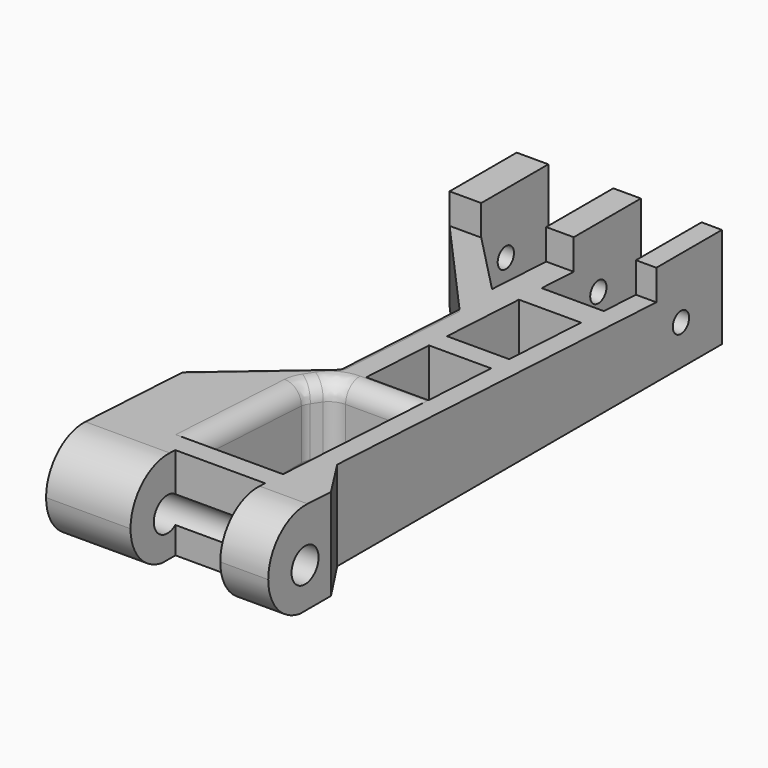
from build123d import *

# Parameters (mm, degrees)
F0_W     = 9.4565711915
F0_H     = 13.6675285175
F1_DEPTH = 15.3
F2_W     = 109.1410517693
F2_H     = 22.5323475897
F3_DEPTH = 77
F4_R     = 2.5676865252
F5_DEPTH = 65.4
F6_R     = 1.5468397632
F7_DEPTH = 54.6
F8_R     = 2.6556349186
F9_R     = 1
F10_R    = 0.0237853743


with BuildPart() as f1:
    # F0 (on Top) → F1 (new body)
    with BuildSketch(Plane.XY):
        Polygon((-40.6965725124, 44.3279668689), (-43.8004508615, 44.3550609052), (-43.8004508615, 25.7457569242), (-53.257022053, 25.7457569242), (-53.257022053, 44.6070879698), (-57.4438385665, 44.6070879698), (-57.4438385665, 21.5618759394), (-67.321151495, 31.8517945707), (-67.321151495, 44.6070879698), (-72.1341744065, 44.6070879698), (-72.1341744065, 31.8517945707), (-57.4438385665, 15.2993714437), (-57.4438385665, -7.5885597616), (-70.2834129333, -20.1490093023), (-70.2834129333, -50.7155247033), (-57.4438385665, -50.7155247033), (-57.4438385665, -38.6135876179), (-43.8004508615, -38.6135876179), (-43.8004508615, -50.7155247033), (-36.5097559988, -50.7155247033), (-36.5097559988, -35.2215506136), (-40.6965725124, -28.8017634302), align=None)
        Polygon((-43.8004508615, -10.5956946412), (-43.8004508615, -35.2215506136), (-57.4438385665, -35.2215506136), (-57.4438385665, -14.0083450824), (-55.5479216548, -10.5956946412), align=None, mode=Mode.SUBTRACT)
        Polygon((-49.6741862581, -7.5885597616), (-53.257022053, -7.5885597616), (-53.257022053, 4.3360902928), (-49.6741862581, 4.3360902928), (-43.8004508615, 4.3360902928), (-43.8004508615, -7.5885597616), align=None, mode=Mode.SUBTRACT)
        with Locations((-48.5287364572, 14.5968659781)):
            Rectangle(F0_W, F0_H, mode=Mode.SUBTRACT)
    extrude(amount=F1_DEPTH)

    # F2 (on face) → F3 (cut)
    with BuildSketch(Plane(origin=(-72.1341744065, 0, 0), x_dir=(0, -1, 0), z_dir=(-1, 0, 0))):
        with Locations((3.7736594677, 6.6085606813)):
            Rectangle(F2_W, F2_H)
        with BuildLine():
            ThreePointArc((39.6816573, 14.1380049634), (44.9345471885, 12.1822751735), (47.1420204778, 7.0301112719))
            ThreePointArc((47.1420204778, 7.0301112719), (44.6510850499, 1.622031227), (38.9221144813, 0))
            Line((38.9221144813, 0), (-31.8517945707, 0))
            Line((-31.8517945707, 0), (-37.1405081916, 0))
            ThreePointArc((-37.1405081916, 0), (-38.2294412702, -0.1143932508), (-39.3183743488, 0))
            Line((-39.3183743488, 0), (-44.6070879698, 0))
            Line((-44.6070879698, 0), (-44.6070879698, 15.3))
            Line((-44.6070879698, 15.3), (-31.8517945707, 15.3))
            Line((-31.8517945707, 15.3), (-31.8517945707, 10.6745666141))
            Line((-31.8517945707, 10.6745666141), (39.6816573, 14.1380049634))
        make_face(mode=Mode.SUBTRACT)
    extrude(amount=-F3_DEPTH, mode=Mode.SUBTRACT)

    # F4 (on face) → F5 (cut)
    with BuildSketch(Plane(origin=(-72.1341744065, 0, 0), x_dir=(0, -1, 0), z_dir=(-1, 0, 0))):
        with Locations((40.1412695646, 6.1273775063)):
            Circle(F4_R)
    extrude(amount=-F5_DEPTH, mode=Mode.SUBTRACT)

    # F6 (on face) → F7 (cut)
    with BuildSketch(Plane(origin=(-72.1341744065, 0, 0), x_dir=(0, -1, 0), z_dir=(-1, 0, 0))):
        with Locations((-36.5287549794, 6.0891942121)):
            Circle(F6_R)
    extrude(amount=-F7_DEPTH, mode=Mode.SUBTRACT)

    # F8
    f8_edges = [f1.edges().sort_by_distance(p)[0] for p in [
        (-56.49588, -12.30202, 0),
        (-55.547922, -10.595695, 6.364874),
        (-56.49588, -12.30202, 12.812364),
        (-57.443839, -14.008345, 6.44749),
        (-49.674186, -10.595695, 0),
        (-57.443839, -24.614948, 0),
        (-49.674186, -10.595695, 12.729749),
        (-57.443839, -24.614948, 13.408519),
    ]]
    fillet(f8_edges, radius=F8_R)

    # F9
    f9_edges = [f1.edges().sort_by_distance(p)[0] for p in [
        (-63.863626, -13.868785, 0),
        (-70.283413, -20.149009, 6.596146),
        (-63.863626, -13.868785, 12.888222),
        (-57.443839, -7.58856, 6.292076),
        (-57.443839, 3.855406, 0),
        (-57.443839, 3.855406, 12.030069),
    ]]
    fillet(f9_edges, radius=F9_R)

    # F10
    f10_edges = [f1.edges().sort_by_distance(p)[0] for p in [
        (-40.696573, 44.327967, 7.65),
        (-43.800451, 44.355061, 7.65),
        (-42.248512, 44.341514, 0),
        (-42.248512, 44.341514, 15.3),
    ]]
    fillet(f10_edges, radius=F10_R)


solid = f1.part
